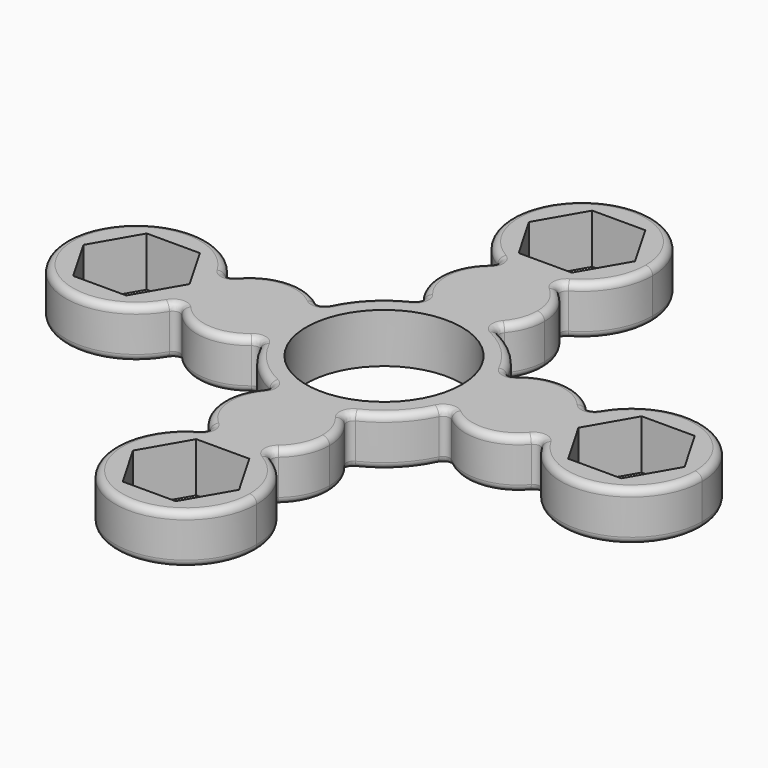
from build123d import *

# Parameters (mm, degrees)
F0_R     = 11
F1_DEPTH = 7
F2_F1_R  = 1
F2_F2_R  = 1


with BuildPart() as f1:
    # F0 (on Top) → F1 (new body)
    with BuildSketch(Plane.XY):
        with BuildLine():
            ThreePointArc((13.1776315789, -4.727581408), (13.7928757354, -2.3992871748), (14, 0))
            ThreePointArc((14, 0), (13.7928757354, 2.3992871748), (13.1776315789, 4.727581408))
            ThreePointArc((13.1776315789, 4.727581408), (11.5, 0), (13.1776315789, -4.727581408))
        make_face()
        with BuildLine():
            ThreePointArc((13.1776315789, 4.727581408), (13.7928757354, 2.3992871748), (14, 0))
            ThreePointArc((14, 0), (13.7928757354, -2.3992871748), (13.1776315789, -4.727581408))
            ThreePointArc((13.1776315789, -4.727581408), (19.7351433448, -7.4638839931), (25.6328125, -3.5008282363))
            ThreePointArc((25.6328125, -3.5008282363), (25, 0), (25.6328125, 3.5008282363))
            ThreePointArc((25.6328125, 3.5008282363), (19.7351433448, 7.4638839931), (13.1776315789, 4.727581408))
        make_face()
        with BuildLine():
            ThreePointArc((13.1776315789, -4.727581408), (11.5, 0), (13.1776315789, 4.727581408))
            ThreePointArc((13.1776315789, 4.727581408), (9.8994949366, 9.8994949366), (4.727581408, 13.1776315789))
            ThreePointArc((4.727581408, 13.1776315789), (0, 11.5), (-4.727581408, 13.1776315789))
            ThreePointArc((-4.727581408, 13.1776315789), (-9.8994949366, 9.8994949366), (-13.1776315789, 4.727581408))
            ThreePointArc((-13.1776315789, 4.727581408), (-11.9318402976, 2.5082102027), (-11.5, 0))
            ThreePointArc((-11.5, 0), (-11.9318402976, -2.5082102027), (-13.1776315789, -4.727581408))
            ThreePointArc((-13.1776315789, -4.727581408), (-9.8994949366, -9.8994949366), (-4.727581408, -13.1776315789))
            ThreePointArc((-4.727581408, -13.1776315789), (0, -11.5), (4.727581408, -13.1776315789))
            ThreePointArc((4.727581408, -13.1776315789), (9.8994949366, -9.8994949366), (13.1776315789, -4.727581408))
        make_face()
        Circle(F0_R, mode=Mode.SUBTRACT)
        with BuildLine():
            ThreePointArc((-4.727581408, 13.1776315789), (0, 11.5), (4.727581408, 13.1776315789))
            ThreePointArc((4.727581408, 13.1776315789), (0, 14), (-4.727581408, 13.1776315789))
        make_face()
        with BuildLine():
            ThreePointArc((-4.727581408, 13.1776315789), (0, 14), (4.727581408, 13.1776315789))
            ThreePointArc((4.727581408, 13.1776315789), (6.7715160991, 15.7756287869), (7.5, 19))
            ThreePointArc((7.5, 19), (6.4228580777, 22.8725823573), (3.5008282363, 25.6328125))
            ThreePointArc((3.5008282363, 25.6328125), (0, 25), (-3.5008282363, 25.6328125))
            ThreePointArc((-3.5008282363, 25.6328125), (-7.4638839931, 19.7351433448), (-4.727581408, 13.1776315789))
        make_face()
        with BuildLine():
            ThreePointArc((45, 0), (36.7787811838, 9.8405252655), (25.6328125, 3.5008282363))
            ThreePointArc((25.6328125, 3.5008282363), (26.2799757469, 1.8033172558), (26.5, 0))
            ThreePointArc((26.5, 0), (26.2799757469, -1.8033172558), (25.6328125, -3.5008282363))
            ThreePointArc((25.6328125, -3.5008282363), (36.7787811838, -9.8405252655), (45, 0))
        make_face()
        Polygon((31.2472232503, -6.5), (27.4944465005, 0), (31.2472232503, 6.5), (38.7527767497, 6.5), (42.5055534995, 0), (38.7527767497, -6.5), align=None, mode=Mode.SUBTRACT)
        with BuildLine():
            ThreePointArc((26.5, 0), (26.2799757469, 1.8033172558), (25.6328125, 3.5008282363))
            ThreePointArc((25.6328125, 3.5008282363), (25, 0), (25.6328125, -3.5008282363))
            ThreePointArc((25.6328125, -3.5008282363), (26.2799757469, -1.8033172558), (26.5, 0))
        make_face()
        with BuildLine():
            ThreePointArc((7.5, -19), (6.7715160991, -15.7756287869), (4.727581408, -13.1776315789))
            ThreePointArc((4.727581408, -13.1776315789), (0, -14), (-4.727581408, -13.1776315789))
            ThreePointArc((-4.727581408, -13.1776315789), (-7.4638839931, -19.7351433448), (-3.5008282363, -25.6328125))
            ThreePointArc((-3.5008282363, -25.6328125), (0, -25), (3.5008282363, -25.6328125))
            ThreePointArc((3.5008282363, -25.6328125), (6.4228580777, -22.8725823573), (7.5, -19))
        make_face()
        with BuildLine():
            ThreePointArc((-4.727581408, -13.1776315789), (0, -14), (4.727581408, -13.1776315789))
            ThreePointArc((4.727581408, -13.1776315789), (0, -11.5), (-4.727581408, -13.1776315789))
        make_face()
        with BuildLine():
            ThreePointArc((-11.5, 0), (-11.9318402976, 2.5082102027), (-13.1776315789, 4.727581408))
            ThreePointArc((-13.1776315789, 4.727581408), (-14, 0), (-13.1776315789, -4.727581408))
            ThreePointArc((-13.1776315789, -4.727581408), (-11.9318402976, -2.5082102027), (-11.5, 0))
        make_face()
        with BuildLine():
            ThreePointArc((-13.1776315789, -4.727581408), (-14, 0), (-13.1776315789, 4.727581408))
            ThreePointArc((-13.1776315789, 4.727581408), (-19.7351433448, 7.4638839931), (-25.6328125, 3.5008282363))
            ThreePointArc((-25.6328125, 3.5008282363), (-25.1594747345, 1.7787811838), (-25, 0))
            ThreePointArc((-25, 0), (-25.1594747345, -1.7787811838), (-25.6328125, -3.5008282363))
            ThreePointArc((-25.6328125, -3.5008282363), (-19.7351433448, -7.4638839931), (-13.1776315789, -4.727581408))
        make_face()
        with BuildLine():
            ThreePointArc((10, 35), (-5.7005139083, 43.216090383), (-3.5008282363, 25.6328125))
            ThreePointArc((-3.5008282363, 25.6328125), (0, 26.5), (3.5008282363, 25.6328125))
            ThreePointArc((3.5008282363, 25.6328125), (8.216090383, 29.2994860917), (10, 35))
        make_face()
        Polygon((7.5055534995, 35), (3.7527767497, 28.5), (-3.7527767497, 28.5), (-7.5055534995, 35), (-3.7527767497, 41.5), (3.7527767497, 41.5), align=None, mode=Mode.SUBTRACT)
        with BuildLine():
            ThreePointArc((3.5008282363, 25.6328125), (0, 26.5), (-3.5008282363, 25.6328125))
            ThreePointArc((-3.5008282363, 25.6328125), (0, 25), (3.5008282363, 25.6328125))
        make_face()
        with BuildLine():
            ThreePointArc((3.5008282363, -25.6328125), (0, -25), (-3.5008282363, -25.6328125))
            ThreePointArc((-3.5008282363, -25.6328125), (0, -26.5), (3.5008282363, -25.6328125))
        make_face()
        with BuildLine():
            ThreePointArc((3.5008282363, -25.6328125), (0, -26.5), (-3.5008282363, -25.6328125))
            ThreePointArc((-3.5008282363, -25.6328125), (-5.7005139083, -43.216090383), (10, -35))
            ThreePointArc((10, -35), (8.216090383, -29.2994860917), (3.5008282363, -25.6328125))
        make_face()
        Polygon((3.7527767497, -28.5), (7.5055534995, -35), (3.7527767497, -41.5), (-3.7527767497, -41.5), (-7.5055534995, -35), (-3.7527767497, -28.5), align=None, mode=Mode.SUBTRACT)
        with BuildLine():
            ThreePointArc((-25, 0), (-25.1594747345, 1.7787811838), (-25.6328125, 3.5008282363))
            ThreePointArc((-25.6328125, 3.5008282363), (-26.5, 0), (-25.6328125, -3.5008282363))
            ThreePointArc((-25.6328125, -3.5008282363), (-25.1594747345, -1.7787811838), (-25, 0))
        make_face()
        with BuildLine():
            ThreePointArc((-25.6328125, -3.5008282363), (-26.5, 0), (-25.6328125, 3.5008282363))
            ThreePointArc((-25.6328125, 3.5008282363), (-45, 0), (-25.6328125, -3.5008282363))
        make_face()
        Polygon((-42.5055534995, 0), (-38.7527767497, 6.5), (-31.2472232503, 6.5), (-27.4944465005, 0), (-31.2472232503, -6.5), (-38.7527767497, -6.5), align=None, mode=Mode.SUBTRACT)
    extrude(amount=F1_DEPTH)

    # F2: fillet of radius 1 on 36 edges, made by hand

    # F2_f1
    f2_f1_edges = [f1.edges().sort_by_distance(p)[0] for p in [
        (-13.1776315789, 4.727581408, 3.5),
        (-25.6328125, 3.5008282363, 3.5),
        (-4.727581408, 13.1776315789, 3.5),
        (-13.1776315789, -4.727581408, 3.5),
        (-4.727581408, -13.1776315789, 3.5),
        (-25.6328125, -3.5008282363, 3.5),
        (4.727581408, -13.1776315789, 3.5),
        (13.1776315789, -4.727581408, 3.5),
        (25.6328125, -3.5008282363, 3.5),
        (25.6328125, 3.5008282363, 3.5),
        (13.1776315789, 4.727581408, 3.5),
        (4.727581408, 13.1776315789, 3.5),
        (-3.5008282363, -25.6328125, 3.5),
        (3.5008282363, -25.6328125, 3.5),
        (3.5008282363, 25.6328125, 3.5),
        (-3.5008282363, 25.6328125, 3.5),
    ]]
    fillet(f2_f1_edges, radius=F2_F1_R)

    # F2_f2
    f2_f2_edges = [f1.edges().sort_by_distance(p)[0] for p in [
        (0, -45, 0),
        (0, -45, 7),
        (0, 45, 0),
        (0, 45, 7),
        (4.5089831044, 25.5666226012, 7),
        (-4.5089831044, 25.5666226012, 7),
        (4.5089831044, 25.5666226012, 0),
        (-4.5089831044, 25.5666226012, 0),
        (-4.5089831044, -25.5666226012, 7),
        (4.5089831044, -25.5666226012, 7),
        (-4.5089831044, -25.5666226012, 0),
        (4.5089831044, -25.5666226012, 0),
    ]]
    fillet(f2_f2_edges, radius=F2_F2_R)


solid = f1.part
